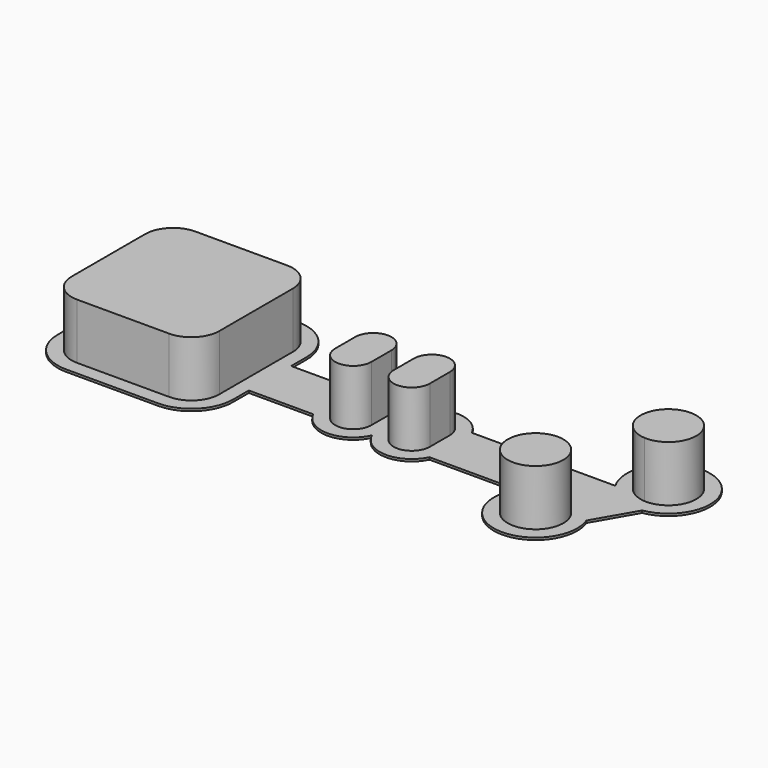
from build123d import *

# Parameters (mm, degrees)
F0_W     = 16
F0_H     = 4.5
F0_W_2   = 6.5
F0_W_3   = 4
F1_DEPTH = 0.4
F2_W     = 6.5
F2_H     = 4.5
F3_DEPTH = 10


# Not quite as in the source:
# - the program builds the solid bodies; features that only make, move or delete a surface that nothing else refers to are left out


with BuildPart() as f1:
    # F0 (on Top) → F1 (new body)
    with BuildSketch(Plane.XY):
        with BuildLine():
            Line((15.75, 4.75), (15.75, 8.25))
            ThreePointArc((15.75, 8.25), (13.5533008589, 13.5533008589), (8.25, 15.75))
            Line((8.25, 15.75), (-8.25, 15.75))
            ThreePointArc((-8.25, 15.75), (-13.5533008589, 13.5533008589), (-15.75, 8.25))
            Line((-15.75, 8.25), (-15.75, -8.25))
            ThreePointArc((-15.75, -8.25), (-13.5533008589, -13.5533008589), (-8.25, -15.75))
            Line((-8.25, -15.75), (8.25, -15.75))
            ThreePointArc((8.25, -15.75), (13.5533008589, -13.5533008589), (15.75, -8.25))
            Line((15.75, -8.25), (15.75, -4.75))
            Line((15.75, -4.75), (27.3219212057, -4.75))
            ThreePointArc((27.3219212057, -4.75), (32.5853423404, -7.9993666334), (37.75, -4.5952078799))
            ThreePointArc((37.75, -4.5952078799), (42.9146576596, -7.9993666334), (48.1780787943, -4.75))
            Line((48.1780787943, -4.75), (63.9480829801, -4.75))
            ThreePointArc((63.9480829801, -4.75), (69.6474451199, -16.1274567319), (77.3637435709, -6.0087617221))
            Line((77.3637435709, -6.0087617221), (81.5596501878, 1.2587617221))
            ThreePointArc((81.5596501878, 1.2587617221), (83.4749132345, 15.4773568118), (73.9480829801, 4.75))
            Line((73.9480829801, 4.75), (48.1780787943, 4.75))
            ThreePointArc((48.1780787943, 4.75), (42.9146576596, 7.9993666334), (37.75, 4.5952078799))
            ThreePointArc((37.75, 4.5952078799), (32.5853423404, 7.9993666334), (27.3219212057, 4.75))
            Line((27.3219212057, 4.75), (15.75, 4.75))
        make_face()
        with BuildLine():
            Line((4.5, 13.25), (8.25, 13.25))
            ThreePointArc((8.25, 13.25), (11.7855339059, 11.7855339059), (13.25, 8.25))
            Line((13.25, 8.25), (13.25, 4.5))
            Line((13.25, 4.5), (13.25, 2.25))
            Line((13.25, 2.25), (29.25, 2.25))
            ThreePointArc((29.25, 2.25), (32.5, 5.5), (35.75, 2.25))
            Line((35.75, 2.25), (39.75, 2.25))
            ThreePointArc((39.75, 2.25), (43, 5.5), (46.25, 2.25))
            Line((46.25, 2.25), (74.0490381057, 2.25))
            Line((74.0490381057, 2.25), (76.1669476654, 5.9183269633))
            ThreePointArc((76.1669476654, 5.9183269633), (82.8480762114, 12.9903810568), (80.0640619824, 3.6683269633))
            Line((80.0640619824, 3.6683269633), (74.5292047573, -5.9183269633))
            ThreePointArc((74.5292047573, -5.9183269633), (69.1116253195, -13.504961376), (67.9923047195, -4.25))
            ThreePointArc((67.9923047195, -4.25), (69.2721438624, -3.7773891431), (70.6320904403, -3.6683269633))
            Line((70.6320904403, -3.6683269633), (71.4509618943, -2.25))
            Line((71.4509618943, -2.25), (46.25, -2.25))
            ThreePointArc((46.25, -2.25), (43, -5.5), (39.75, -2.25))
            Line((39.75, -2.25), (35.75, -2.25))
            ThreePointArc((35.75, -2.25), (32.5, -5.5), (29.25, -2.25))
            Line((29.25, -2.25), (13.25, -2.25))
            Line((13.25, -2.25), (13.25, -4.5))
            Line((13.25, -4.5), (13.25, -8.25))
            ThreePointArc((13.25, -8.25), (11.7855339059, -11.7855339059), (8.25, -13.25))
            Line((8.25, -13.25), (4.5, -13.25))
            Line((4.5, -13.25), (-4.5, -13.25))
            Line((-4.5, -13.25), (-8.25, -13.25))
            ThreePointArc((-8.25, -13.25), (-11.7855339059, -11.7855339059), (-13.25, -8.25))
            Line((-13.25, -8.25), (-13.25, -4.5))
            Line((-13.25, -4.5), (-13.25, 4.5))
            Line((-13.25, 4.5), (-13.25, 8.25))
            ThreePointArc((-13.25, 8.25), (-11.7855339059, 11.7855339059), (-8.25, 13.25))
            Line((-8.25, 13.25), (-4.5, 13.25))
            Line((-4.5, 13.25), (4.5, 13.25))
        make_face(mode=Mode.SUBTRACT)
        with BuildLine():
            Line((13.25, -4.5), (4.5, -4.5))
            Line((4.5, -4.5), (4.5, -13.25))
            Line((4.5, -13.25), (8.25, -13.25))
            ThreePointArc((8.25, -13.25), (11.7855339059, -11.7855339059), (13.25, -8.25))
            Line((13.25, -8.25), (13.25, -4.5))
        make_face()
        Polygon((13.25, 4.5), (4.5, 4.5), (4.5, 0), (4.5, -4.5), (13.25, -4.5), (13.25, -2.25), (13.25, 2.25), align=None)
        with BuildLine():
            ThreePointArc((13.25, 8.25), (11.7855339059, 11.7855339059), (8.25, 13.25))
            Line((8.25, 13.25), (4.5, 13.25))
            Line((4.5, 13.25), (4.5, 4.5))
            Line((4.5, 4.5), (13.25, 4.5))
            Line((13.25, 4.5), (13.25, 8.25))
        make_face()
        Polygon((4.5, 4.5), (4.5, 13.25), (-4.5, 13.25), (-4.5, 4.5), (0, 4.5), align=None)
        with Locations((21.25, 0)):
            Rectangle(F0_W, F0_H)
        with Locations((32.5, 0)):
            Rectangle(F0_W_2, F0_H)
        with BuildLine():
            ThreePointArc((35.75, 2.25), (32.5, 5.5), (29.25, 2.25))
            Line((29.25, 2.25), (35.75, 2.25))
        make_face()
        with BuildLine():
            Line((35.75, -2.25), (29.25, -2.25))
            ThreePointArc((29.25, -2.25), (32.5, -5.5), (35.75, -2.25))
        make_face()
        with Locations((37.75, 0)):
            Rectangle(F0_W_3, F0_H)
        with BuildLine():
            ThreePointArc((46.25, 2.25), (43, 5.5), (39.75, 2.25))
            Line((39.75, 2.25), (46.25, 2.25))
        make_face()
        with Locations((43, 0)):
            Rectangle(F0_W_2, F0_H)
        with BuildLine():
            Line((46.25, -2.25), (39.75, -2.25))
            ThreePointArc((39.75, -2.25), (43, -5.5), (46.25, -2.25))
        make_face()
        Polygon((74.0490381057, 2.25), (46.25, 2.25), (46.25, -2.25), (71.4509618943, -2.25), align=None)
        with BuildLine():
            ThreePointArc((80.0640619824, 3.6683269633), (82.8480762114, 12.9903810568), (76.1669476654, 5.9183269633))
            ThreePointArc((76.1669476654, 5.9183269633), (77.8480762114, 4.3301270189), (80.0640619824, 3.6683269633))
        make_face()
        with BuildLine():
            Line((76.1669476654, 5.9183269633), (74.0490381057, 2.25))
            Line((74.0490381057, 2.25), (71.4509618943, -2.25))
            Line((71.4509618943, -2.25), (70.6320904403, -3.6683269633))
            ThreePointArc((70.6320904403, -3.6683269633), (72.8480762114, -4.3301270189), (74.5292047573, -5.9183269633))
            Line((74.5292047573, -5.9183269633), (80.0640619824, 3.6683269633))
            ThreePointArc((80.0640619824, 3.6683269633), (77.8480762114, 4.3301270189), (76.1669476654, 5.9183269633))
        make_face()
        with BuildLine():
            ThreePointArc((74.5292047573, -5.9183269633), (72.8480762114, -4.3301270189), (70.6320904403, -3.6683269633))
            ThreePointArc((70.6320904403, -3.6683269633), (69.2721438624, -3.7773891431), (67.9923047195, -4.25))
            ThreePointArc((67.9923047195, -4.25), (69.1116253195, -13.504961376), (74.5292047573, -5.9183269633))
        make_face()
        Polygon((4.5, -4.5), (0, -4.5), (-4.5, -4.5), (-4.5, -13.25), (4.5, -13.25), align=None)
        with BuildLine():
            ThreePointArc((0, -4.5), (3.1819805153, -3.1819805153), (4.5, 0))
            ThreePointArc((4.5, 0), (3.1819805153, 3.1819805153), (0, 4.5))
            ThreePointArc((0, 4.5), (-3.1819805153, 3.1819805153), (-4.5, 0))
            ThreePointArc((-4.5, 0), (-3.1819805153, -3.1819805153), (0, -4.5))
        make_face()
        with BuildLine():
            Line((-4.5, -13.25), (-4.5, -4.5))
            Line((-4.5, -4.5), (-13.25, -4.5))
            Line((-13.25, -4.5), (-13.25, -8.25))
            ThreePointArc((-13.25, -8.25), (-11.7855339059, -11.7855339059), (-8.25, -13.25))
            Line((-8.25, -13.25), (-4.5, -13.25))
        make_face()
        Polygon((-4.5, 0), (-4.5, 4.5), (-13.25, 4.5), (-13.25, -4.5), (-4.5, -4.5), align=None)
        with BuildLine():
            Line((-4.5, 4.5), (-4.5, 13.25))
            Line((-4.5, 13.25), (-8.25, 13.25))
            ThreePointArc((-8.25, 13.25), (-11.7855339059, 11.7855339059), (-13.25, 8.25))
            Line((-13.25, 8.25), (-13.25, 4.5))
            Line((-13.25, 4.5), (-4.5, 4.5))
        make_face()
        with BuildLine():
            Line((4.5, 0), (4.5, 4.5))
            Line((4.5, 4.5), (0, 4.5))
            ThreePointArc((0, 4.5), (3.1819805153, 3.1819805153), (4.5, 0))
        make_face()
        with BuildLine():
            Line((4.5, -4.5), (4.5, 0))
            ThreePointArc((4.5, 0), (3.1819805153, -3.1819805153), (0, -4.5))
            Line((0, -4.5), (4.5, -4.5))
        make_face()
        with BuildLine():
            ThreePointArc((0, -4.5), (-3.1819805153, -3.1819805153), (-4.5, 0))
            Line((-4.5, 0), (-4.5, -4.5))
            Line((-4.5, -4.5), (0, -4.5))
        make_face()
        with BuildLine():
            Line((0, 4.5), (-4.5, 4.5))
            Line((-4.5, 4.5), (-4.5, 0))
            ThreePointArc((-4.5, 0), (-3.1819805153, 3.1819805153), (0, 4.5))
        make_face()
    extrude(amount=F1_DEPTH)

    # F2 (on face) → F3 (join)
    with BuildSketch(Plane.XY.offset(0.4)):
        with BuildLine():
            Line((-4.5, 4.5), (-4.5, 13.25))
            Line((-4.5, 13.25), (-8.25, 13.25))
            ThreePointArc((-8.25, 13.25), (-11.7855339059, 11.7855339059), (-13.25, 8.25))
            Line((-13.25, 8.25), (-13.25, 4.5))
            Line((-13.25, 4.5), (-4.5, 4.5))
        make_face()
        Polygon((4.5, 4.5), (4.5, 13.25), (-4.5, 13.25), (-4.5, 4.5), (0, 4.5), align=None)
        with BuildLine():
            ThreePointArc((13.25, 8.25), (11.7855339059, 11.7855339059), (8.25, 13.25))
            Line((8.25, 13.25), (4.5, 13.25))
            Line((4.5, 13.25), (4.5, 4.5))
            Line((4.5, 4.5), (13.25, 4.5))
            Line((13.25, 4.5), (13.25, 8.25))
        make_face()
        Polygon((13.25, 4.5), (4.5, 4.5), (4.5, 0), (4.5, -4.5), (13.25, -4.5), (13.25, -2.25), (13.25, 2.25), align=None)
        Polygon((4.5, -4.5), (0, -4.5), (-4.5, -4.5), (-4.5, -13.25), (4.5, -13.25), align=None)
        with BuildLine():
            Line((-4.5, -13.25), (-4.5, -4.5))
            Line((-4.5, -4.5), (-13.25, -4.5))
            Line((-13.25, -4.5), (-13.25, -8.25))
            ThreePointArc((-13.25, -8.25), (-11.7855339059, -11.7855339059), (-8.25, -13.25))
            Line((-8.25, -13.25), (-4.5, -13.25))
        make_face()
        Polygon((-4.5, 0), (-4.5, 4.5), (-13.25, 4.5), (-13.25, -4.5), (-4.5, -4.5), align=None)
        with BuildLine():
            ThreePointArc((0, -4.5), (3.1819805153, -3.1819805153), (4.5, 0))
            ThreePointArc((4.5, 0), (3.1819805153, 3.1819805153), (0, 4.5))
            ThreePointArc((0, 4.5), (-3.1819805153, 3.1819805153), (-4.5, 0))
            ThreePointArc((-4.5, 0), (-3.1819805153, -3.1819805153), (0, -4.5))
        make_face()
        with BuildLine():
            Line((4.5, 0), (4.5, 4.5))
            Line((4.5, 4.5), (0, 4.5))
            ThreePointArc((0, 4.5), (3.1819805153, 3.1819805153), (4.5, 0))
        make_face()
        with BuildLine():
            Line((0, 4.5), (-4.5, 4.5))
            Line((-4.5, 4.5), (-4.5, 0))
            ThreePointArc((-4.5, 0), (-3.1819805153, 3.1819805153), (0, 4.5))
        make_face()
        with BuildLine():
            ThreePointArc((0, -4.5), (-3.1819805153, -3.1819805153), (-4.5, 0))
            Line((-4.5, 0), (-4.5, -4.5))
            Line((-4.5, -4.5), (0, -4.5))
        make_face()
        with BuildLine():
            Line((4.5, -4.5), (4.5, 0))
            ThreePointArc((4.5, 0), (3.1819805153, -3.1819805153), (0, -4.5))
            Line((0, -4.5), (4.5, -4.5))
        make_face()
        with BuildLine():
            Line((13.25, -4.5), (4.5, -4.5))
            Line((4.5, -4.5), (4.5, -13.25))
            Line((4.5, -13.25), (8.25, -13.25))
            ThreePointArc((8.25, -13.25), (11.7855339059, -11.7855339059), (13.25, -8.25))
            Line((13.25, -8.25), (13.25, -4.5))
        make_face()
        with BuildLine():
            ThreePointArc((35.75, 2.25), (32.5, 5.5), (29.25, 2.25))
            Line((29.25, 2.25), (35.75, 2.25))
        make_face()
        with Locations((32.5, 0)):
            Rectangle(F2_W, F2_H)
        with BuildLine():
            Line((35.75, -2.25), (29.25, -2.25))
            ThreePointArc((29.25, -2.25), (32.5, -5.5), (35.75, -2.25))
        make_face()
        with BuildLine():
            ThreePointArc((46.25, 2.25), (43, 5.5), (39.75, 2.25))
            Line((39.75, 2.25), (46.25, 2.25))
        make_face()
        with Locations((43, 0)):
            Rectangle(F2_W, F2_H)
        with BuildLine():
            Line((46.25, -2.25), (39.75, -2.25))
            ThreePointArc((39.75, -2.25), (43, -5.5), (46.25, -2.25))
        make_face()
        with BuildLine():
            ThreePointArc((72.8480762114, -4.3301270189), (71.7788727151, -3.8693437522), (70.6320904403, -3.6683269633))
            ThreePointArc((70.6320904403, -3.6683269633), (67.8480762114, -12.9903810568), (74.5292047573, -5.9183269633))
            ThreePointArc((74.5292047573, -5.9183269633), (73.7817279741, -5.0256927751), (72.8480762114, -4.3301270189))
        make_face()
        with BuildLine():
            ThreePointArc((80.0640619824, 3.6683269633), (82.8480762114, 12.9903810568), (76.1669476654, 5.9183269633))
            ThreePointArc((76.1669476654, 5.9183269633), (76.9144244486, 5.0256927751), (77.8480762114, 4.3301270189))
            ThreePointArc((77.8480762114, 4.3301270189), (78.9172797076, 3.8693437522), (80.0640619824, 3.6683269633))
        make_face()
    extrude(amount=F3_DEPTH)


solid = f1.part
